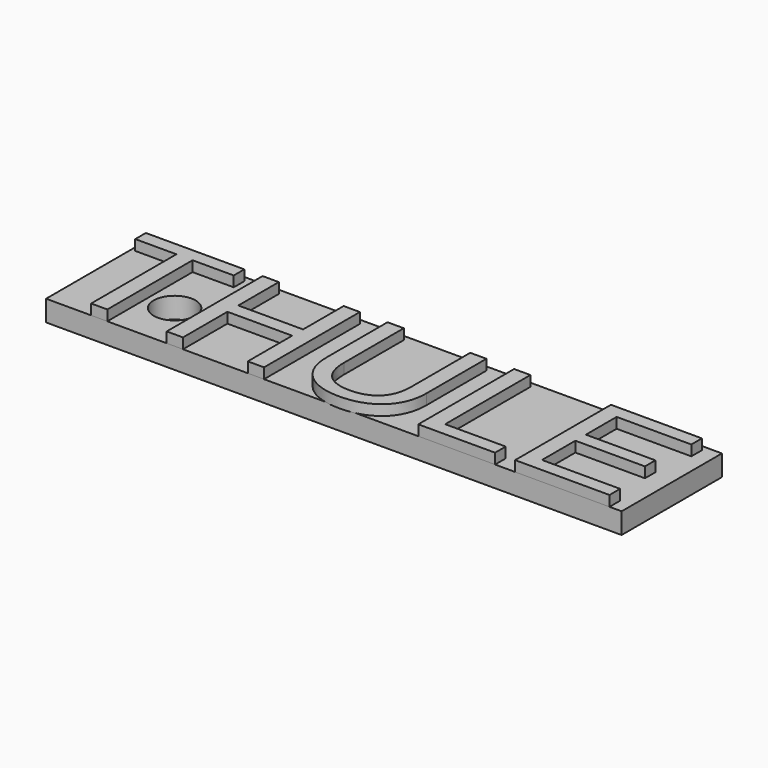
from build123d import *

# Parameters (mm, degrees)
F0_TEXT_SIZE = 16.6666666667
F2_DEPTH     = 1
F1_W         = 55.078125
F1_H         = 12
F3_DEPTH     = 2
F4_R         = 2
F5_DEPTH     = 2.001


# Not quite as in the source:
# - Text() gives the source's letters only with a copy of the font that has no kerning and outlines rounded to 1/6400 em; it was checked with that copy


with BuildPart() as f2:
    # F0 (on Top) → F2 (new body)
    with BuildSketch(Plane.XY):
        with Locations((-40.9701470463, 0)):
            Text('THULE', F0_TEXT_SIZE, font='Arimo', text_align=(TextAlign.LEFT, TextAlign.BOTTOM))
    extrude(amount=F2_DEPTH)


with BuildPart() as f3:
    # F1 (on Top) → F3 (new body)
    with BuildSketch(Plane.XY):
        with Locations((-13.4310845463, 6)):
            Rectangle(F1_W, F1_H)
    extrude(amount=-F3_DEPTH)

    # F4 (on face) → F5 (cut, through all)
    with BuildSketch(Plane.XY):
        with Locations((-32.520595938, 4.8137959093)):
            Circle(F4_R)
    extrude(amount=-F5_DEPTH, mode=Mode.SUBTRACT)


solid = Compound([f2.part, f3.part])
